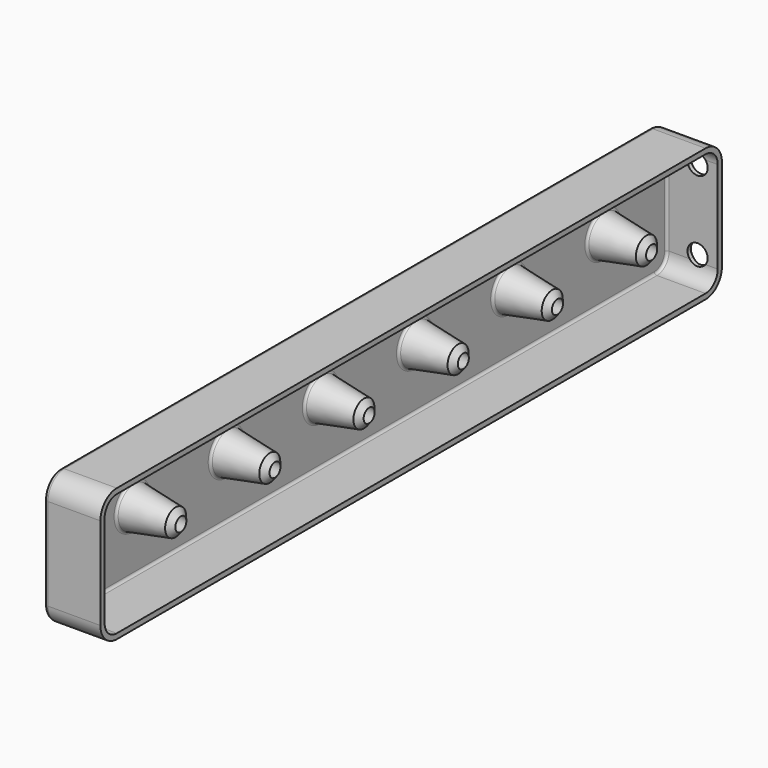
from build123d import *

# Parameters (mm, degrees)
F0_W         = 915
F0_H         = 165.1
F1_DEPTH     = 70
F2_DEPTH     = 36.63
F3_DEPTH     = 12.5
F4_R         = 20.32
F5_DEPTH     = 70.001
F5_TAPER     = 10
F6_R         = 5
F7_T1_DEPTH  = 133.5
F7_T4_ANGLE  = 90
F7_T6_ANGLE  = 90
F7_T8_ANGLE  = 90
F7_T10_ANGLE = 90
F8_T         = -6.5
F9_R         = 3.175
F12_DEPTH    = 25
F13_R        = 2


# Not quite as in the source:
# - a fillet or chamfer that OpenCascade refuses, or shapes differently, is made with other operations: its cross-section is extruded or revolved along the edge and cut away or added


with BuildPart() as f1:
    # F0 (on Right) → F1 (new body)
    with BuildSketch(Plane.YZ):
        Rectangle(F0_W, F0_H)
    extrude(amount=F1_DEPTH)

    # F2 (add): a face of the model
    f2_faces = [f1.faces().sort_by_distance(p)[0] for p in [
        (35, -457.5, 0),
    ]]
    extrude(f2_faces, amount=F2_DEPTH)

    # F3 (add): a face of the model
    f3_faces = [f1.faces().sort_by_distance(p)[0] for p in [
        (35, 457.5, 0),
    ]]
    extrude(f3_faces, amount=F3_DEPTH)

    # F4 (on face) → F5 (cut, through all)
    with BuildSketch(Plane.YZ):
        with Locations((-365.125, 0)):
            Circle(F4_R)
        with Locations((-73.025, 0)):
            Circle(F4_R)
        with Locations((73.025, 0)):
            Circle(F4_R)
        with Locations((-219.075, 0)):
            Circle(F4_R)
        with Locations((219.075, 0)):
            Circle(F4_R)
        with Locations((365.125, 0)):
            Circle(F4_R)
    extrude(amount=F5_DEPTH, taper=F5_TAPER, mode=Mode.SUBTRACT)

    # F6
    f6_edges = [f1.edges().sort_by_distance(p)[0] for p in [
        (0, -494.13, 0),
        (0, -12.065, 82.55),
        (0, -12.065, -82.55),
        (0, 470, 0),
        (0, -385.445, 0),
        (0, -239.395, 0),
        (0, -93.345, 0),
        (0, 52.705, 0),
        (0, 198.755, 0),
        (0, 344.805, 0),
    ]]
    fillet(f6_edges, radius=F6_R)

    # F7: fillet of radius 25.4 on 4 edges, made by hand

    # F7_s2 → F7_t1 (cut)
    with BuildSketch(Plane.YZ):
        with BuildLine():
            ThreePointArc((-468.73, 82.55), (-486.6905122421, 75.1105122421), (-494.13, 57.15))
            Line((-494.13, 57.15), (-494.13, 82.55))
            Line((-494.13, 82.55), (-468.73, 82.55))
        make_face()
        with BuildLine():
            ThreePointArc((-494.13, -57.15), (-486.6905122421, -75.1105122421), (-468.73, -82.55))
            Line((-468.73, -82.55), (-494.13, -82.55))
            Line((-494.13, -82.55), (-494.13, -57.15))
        make_face()
        with BuildLine():
            ThreePointArc((470, -57.15), (462.5605122421, -75.1105122421), (444.6, -82.55))
            Line((444.6, -82.55), (470, -82.55))
            Line((470, -82.55), (470, -57.15))
        make_face()
        with BuildLine():
            ThreePointArc((444.6, 82.55), (462.5605122421, 75.1105122421), (470, 57.15))
            Line((470, 57.15), (470, 82.55))
            Line((470, 82.55), (444.6, 82.55))
        make_face()
    extrude(amount=F7_T1_DEPTH, mode=Mode.SUBTRACT)

    # F7_s3 → F7_t4 (revolve, cut)
    with BuildSketch(Plane.XZ.offset(-444.6)):
        with BuildLine():
            ThreePointArc((0, 77.55), (1.4644660941, 81.0855339059), (5, 82.55))
            Line((5, 82.55), (0, 82.55))
            Line((0, 82.55), (0, 77.55))
        make_face()
    revolve(axis=Axis((0, 444.6, 57.15), (-1, 0, 0)), revolution_arc=F7_T4_ANGLE, mode=Mode.SUBTRACT)

    # F7_s5 → F7_t6 (revolve, cut)
    with BuildSketch(Plane.XY.offset(-57.15)):
        with BuildLine():
            ThreePointArc((0, 465), (1.4644660941, 468.5355339059), (5, 470))
            Line((5, 470), (0, 470))
            Line((0, 470), (0, 465))
        make_face()
    revolve(axis=Axis((0, 444.6, -57.15), (-1, 0, 0)), revolution_arc=F7_T6_ANGLE, mode=Mode.SUBTRACT)

    # F7_s7 → F7_t8 (revolve, cut)
    with BuildSketch(Plane.XZ.offset(468.73)):
        with BuildLine():
            ThreePointArc((0, -77.55), (1.4644660941, -81.0855339059), (5, -82.55))
            Line((5, -82.55), (0, -82.55))
            Line((0, -82.55), (0, -77.55))
        make_face()
    revolve(axis=Axis((0, -468.73, -57.15), (-1, 0, 0)), revolution_arc=F7_T8_ANGLE, mode=Mode.SUBTRACT)

    # F7_s9 → F7_t10 (revolve, cut)
    with BuildSketch(Plane.XY.offset(57.15)):
        with BuildLine():
            ThreePointArc((0, -489.13), (1.4644660941, -492.6655339059), (5, -494.13))
            Line((5, -494.13), (0, -494.13))
            Line((0, -494.13), (0, -489.13))
        make_face()
    revolve(axis=Axis((0, -468.73, 57.15), (-1, 0, 0)), revolution_arc=F7_T10_ANGLE, mode=Mode.SUBTRACT)

    # F8
    f8_openings = [f1.faces().sort_by_distance(p)[0] for p in [
        (70, -12.156928, 0),
    ]]
    offset(amount=F8_T, openings=f8_openings, kind=Kind.INTERSECTION)

    # F9
    f9_edges = [f1.edges().sort_by_distance(p)[0] for p in [
        (6.5, 339.350852, 0),
        (6.5, -390.899148, 0),
        (6.5, -12.065, -76.05),
        (6.5, 457.964318, -70.514318),
        (6.5, 463.5, 0),
        (6.5, 457.964318, 70.514318),
        (6.5, -12.065, 76.05),
        (6.5, -482.094318, 70.514318),
        (6.5, -487.63, 0),
        (6.5, -482.094318, -70.514318),
        (6.5, 193.300852, 0),
        (6.5, 47.250852, 0),
        (6.5, -98.799148, 0),
        (6.5, -244.849148, 0),
    ]]
    fillet(f9_edges, radius=F9_R)

    # F10: chamfer of 10 on 6 edges, made by hand

    # F10_s1 → F10_t2 (revolve, cut)
    with BuildSketch(Plane.XY):
        Polygon((60.1519224699, 381.4388661043), (70, 369.7023843277), (70, 379.7023843277), align=None)
    revolve(axis=Axis((70, 365.125, 0), (1, 0, 0)), mode=Mode.SUBTRACT)

    # F10_s3 → F10_t4 (revolve, cut)
    with BuildSketch(Plane.XY):
        Polygon((60.1519224699, -348.8111338957), (70, -360.5476156723), (70, -350.5476156723), align=None)
    revolve(axis=Axis((70, -365.125, 0), (1, 0, 0)), mode=Mode.SUBTRACT)

    # F10_s5 → F10_t6 (revolve, cut)
    with BuildSketch(Plane.XY):
        Polygon((60.1519224699, 235.3888661043), (70, 223.6523843277), (70, 233.6523843277), align=None)
    revolve(axis=Axis((70, 219.075, 0), (1, 0, 0)), mode=Mode.SUBTRACT)

    # F10_s7 → F10_t8 (revolve, cut)
    with BuildSketch(Plane.XY):
        Polygon((60.1519224699, 89.3388661043), (70, 77.6023843277), (70, 87.6023843277), align=None)
    revolve(axis=Axis((70, 73.025, 0), (1, 0, 0)), mode=Mode.SUBTRACT)

    # F10_s9 → F10_t10 (revolve, cut)
    with BuildSketch(Plane.XY):
        Polygon((60.1519224699, -56.7111338957), (70, -68.4476156723), (70, -58.4476156723), align=None)
    revolve(axis=Axis((70, -73.025, 0), (1, 0, 0)), mode=Mode.SUBTRACT)

    # F10_s11 → F10_t12 (revolve, cut)
    with BuildSketch(Plane.XY):
        Polygon((60.1519224699, -202.7611338957), (70, -214.4976156723), (70, -204.4976156723), align=None)
    revolve(axis=Axis((70, -219.075, 0), (1, 0, 0)), mode=Mode.SUBTRACT)

    # F11 (on face) → F12 (cut)
    with BuildSketch(Plane(origin=(0, 470, 0), x_dir=(-1, 0, 0), z_dir=(0, 1, 0))):
        with BuildLine():
            Line((-54.807522623, 57.15), (-35.192477377, 57.15))
            ThreePointArc((-35.192477377, 57.15), (-45, 61.9), (-54.807522623, 57.15))
        make_face()
        with BuildLine():
            ThreePointArc((-54.807522623, 57.15), (-49.1021925365, 37.5922899598), (-32.5, 49.4))
            ThreePointArc((-32.5, 49.4), (-33.1922899598, 53.5021925365), (-35.192477377, 57.15))
            Line((-35.192477377, 57.15), (-54.807522623, 57.15))
        make_face()
        with BuildLine():
            Line((-54.807522623, -57.15), (-35.192477377, -57.15))
            ThreePointArc((-35.192477377, -57.15), (-33.1922899598, -53.5021925365), (-32.5, -49.4))
            ThreePointArc((-32.5, -49.4), (-49.1021925365, -37.5922899598), (-54.807522623, -57.15))
        make_face()
        with BuildLine():
            ThreePointArc((-54.807522623, -57.15), (-45, -61.9), (-35.192477377, -57.15))
            Line((-35.192477377, -57.15), (-54.807522623, -57.15))
        make_face()
    extrude(amount=-F12_DEPTH, mode=Mode.SUBTRACT)

    # F13
    f13_edges = [f1.edges().sort_by_distance(p)[0] for p in [
        (45, 469.551904, 61.9),
        (45, 470, 36.9),
        (45, 470, -36.9),
        (44.999991, 469.551904, -61.9),
    ]]
    fillet(f13_edges, radius=F13_R)


solid = f1.part
